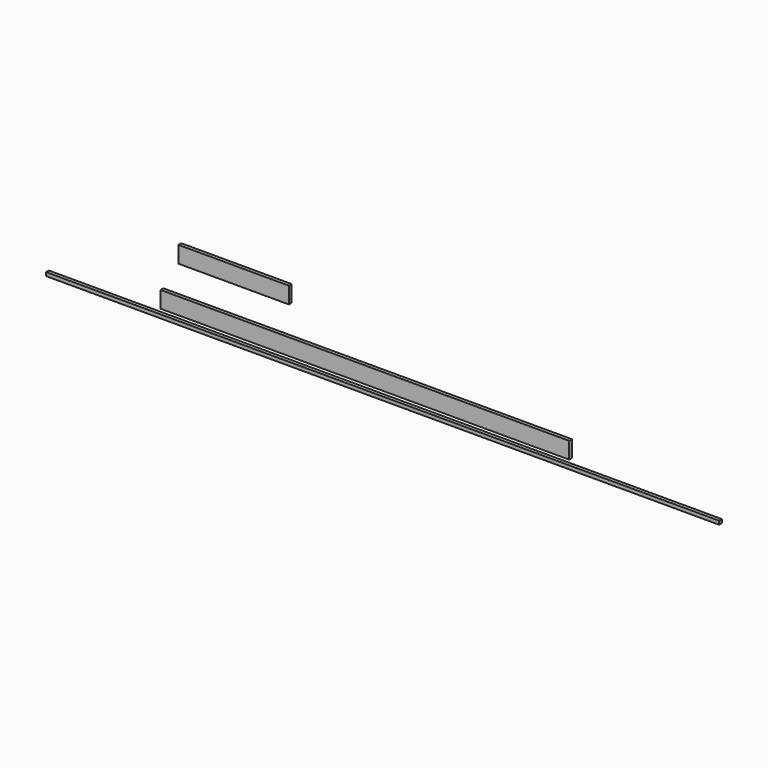
from build123d import *

# Parameters (mm, degrees)
F1_E0_TOP_W = 3047.2222391173
F1_E0_TOP_H = 16
F3_DEPTH    = 16
F6_W        = 1850
F6_H        = 75
F7_DEPTH    = 16
F8_W        = 500
F8_H        = 75
F9_DEPTH    = 16


# Not quite as in the source:
# - the program builds the solid bodies; features that only make, move or delete a surface that nothing else refers to are left out


with BuildPart() as f3:
    # F1_E0_top (on explicit) → F3 (new body)
    with BuildSketch(Plane(origin=(-1523.3105482362, 0, -29.0839689784), x_dir=(1, 0, 0), z_dir=(0, 0, -1))):
        with Locations((1523.6111195587, 8)):
            Rectangle(F1_E0_TOP_W, F1_E0_TOP_H)
    extrude(amount=F3_DEPTH)


with BuildPart() as f7:
    # F6 (on Front) → F7 (new body)
    with BuildSketch(Plane.XZ):
        with Locations((-79.9069583416, 31.0795101923)):
            Rectangle(F6_W, F6_H)
    extrude(amount=F7_DEPTH)


with BuildPart() as f9:
    # F8 (on face) → F9 (new body)
    with BuildSketch(Plane.XZ.offset(16)):
        with Locations((-661.014303565, 247.5882079988)):
            Rectangle(F8_W, F8_H)
    extrude(amount=F9_DEPTH)


solid = Compound([f3.part, f7.part, f9.part])
